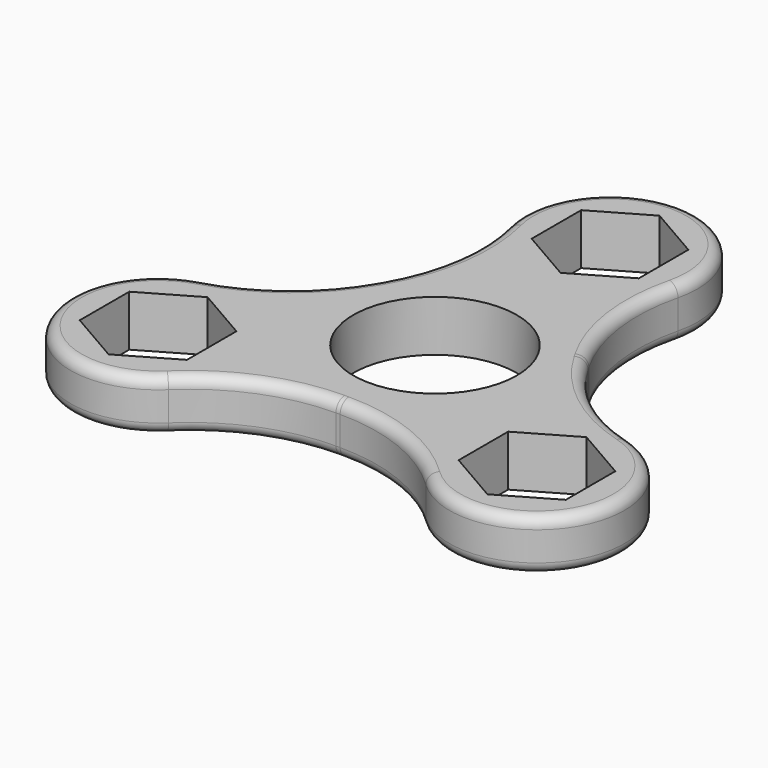
from build123d import *

# Parameters (mm, degrees)
F0_R     = 11.225
F1_DEPTH = 7
F2_R     = 25
F3_R     = 1.5


with BuildPart() as f1:
    # F0 (on Top) → F1 (new body)
    with BuildSketch(Plane.XY):
        with BuildLine():
            Line((-14.0909507949, -16.6224631917), (-8.8518149883, -13.5976467234))
            ThreePointArc((-8.8518149883, -13.5976467234), (0, -16.225), (8.8518149883, -13.5976467234))
            Line((8.8518149883, -13.5976467234), (14.0909507949, -16.6224631917))
            ThreePointArc((14.0909507949, -16.6224631917), (36.3730669589, -21), (21.4409507949, -3.8918897561))
            Line((21.4409507949, -3.8918897561), (16.2018149883, -0.8670732877))
            ThreePointArc((16.2018149883, -0.8670732877), (14.0512621764, 8.1125), (7.35, 14.4647200111))
            Line((7.35, 14.4647200111), (7.35, 20.5143529477))
            ThreePointArc((7.35, 20.5143529477), (0, 42), (-7.35, 20.5143529477))
            Line((-7.35, 20.5143529477), (-7.35, 14.4647200111))
            ThreePointArc((-7.35, 14.4647200111), (-14.0512621764, 8.1125), (-16.2018149883, -0.8670732877))
            Line((-16.2018149883, -0.8670732877), (-21.4409507949, -3.8918897561))
            ThreePointArc((-21.4409507949, -3.8918897561), (-36.3730669589, -21), (-14.0909507949, -16.6224631917))
        make_face()
        Polygon((-25.9807621135, -23.4870489571), (-33.3307621135, -19.2435244785), (-33.3307621135, -10.7564755215), (-25.9807621135, -6.5129510429), (-18.6307621135, -10.7564755215), (-18.6307621135, -19.2435244785), align=None, mode=Mode.SUBTRACT)
        Circle(F0_R, mode=Mode.SUBTRACT)
        Polygon((33.3307621135, -10.7564755215), (33.3307621135, -19.2435244785), (25.9807621135, -23.4870489571), (18.6307621135, -19.2435244785), (18.6307621135, -10.7564755215), (25.9807621135, -6.5129510429), align=None, mode=Mode.SUBTRACT)
        Polygon((0, 38.4870489571), (7.35, 34.2435244785), (7.35, 25.7564755215), (0, 21.5129510429), (-7.35, 25.7564755215), (-7.35, 34.2435244785), align=None, mode=Mode.SUBTRACT)
        with BuildLine():
            Line((-7.35, 20.5143529477), (-21.4409507949, -3.8918897561))
            Line((-21.4409507949, -3.8918897561), (-16.2018149883, -0.8670732877))
            ThreePointArc((-16.2018149883, -0.8670732877), (-14.0512621764, 8.1125), (-7.35, 14.4647200111))
            Line((-7.35, 14.4647200111), (-7.35, 20.5143529477))
        make_face()
        with BuildLine():
            Line((16.2018149883, -0.8670732877), (21.4409507949, -3.8918897561))
            Line((21.4409507949, -3.8918897561), (7.35, 20.5143529477))
            Line((7.35, 20.5143529477), (7.35, 14.4647200111))
            ThreePointArc((7.35, 14.4647200111), (14.0512621764, 8.1125), (16.2018149883, -0.8670732877))
        make_face()
        with BuildLine():
            ThreePointArc((8.8518149883, -13.5976467234), (0, -16.225), (-8.8518149883, -13.5976467234))
            Line((-8.8518149883, -13.5976467234), (-14.0909507949, -16.6224631917))
            Line((-14.0909507949, -16.6224631917), (14.0909507949, -16.6224631917))
            Line((14.0909507949, -16.6224631917), (8.8518149883, -13.5976467234))
        make_face()
    extrude(amount=F1_DEPTH)

    # F2
    f2_edges = [f1.edges().sort_by_distance(p)[0] for p in [
        (-21.440951, -3.89189, 3.5),
        (7.35, 20.514353, 3.5),
        (14.090951, -16.622463, 3.5),
        (21.440951, -3.89189, 3.5),
        (-7.35, 20.514353, 3.5),
        (-14.090951, -16.622463, 3.5),
    ]]
    fillet(f2_edges, radius=F2_R)

    # F3
    f3_edges = [f1.edges().sort_by_distance(p)[0] for p in [
        (-11.147106, 17.57587, 7),
        (-20.794703, 0.865742, 7),
        (-36.373067, -21, 7),
        (-9.647597, -18.441612, 7),
        (36.373067, -21, 7),
        (20.794703, 0.865742, 7),
        (11.147106, 17.57587, 7),
        (0, 42, 7),
        (0, 42, 0),
        (-11.147106, 17.57587, 0),
        (-20.794703, 0.865742, 0),
        (-36.373067, -21, 0),
        (-9.647597, -18.441612, 0),
        (9.647597, -18.441612, 0),
        (36.373067, -21, 0),
        (20.794703, 0.865742, 0),
        (0, -16.622463, 0),
        (14.395475, 8.311232, 0),
        (11.147106, 17.57587, 0),
        (-14.395475, 8.311232, 0),
        (9.647597, -18.441612, 7),
        (0, -16.622463, 7),
        (14.395475, 8.311232, 7),
        (-14.395475, 8.311232, 7),
    ]]
    fillet(f3_edges, radius=F3_R)


solid = f1.part
